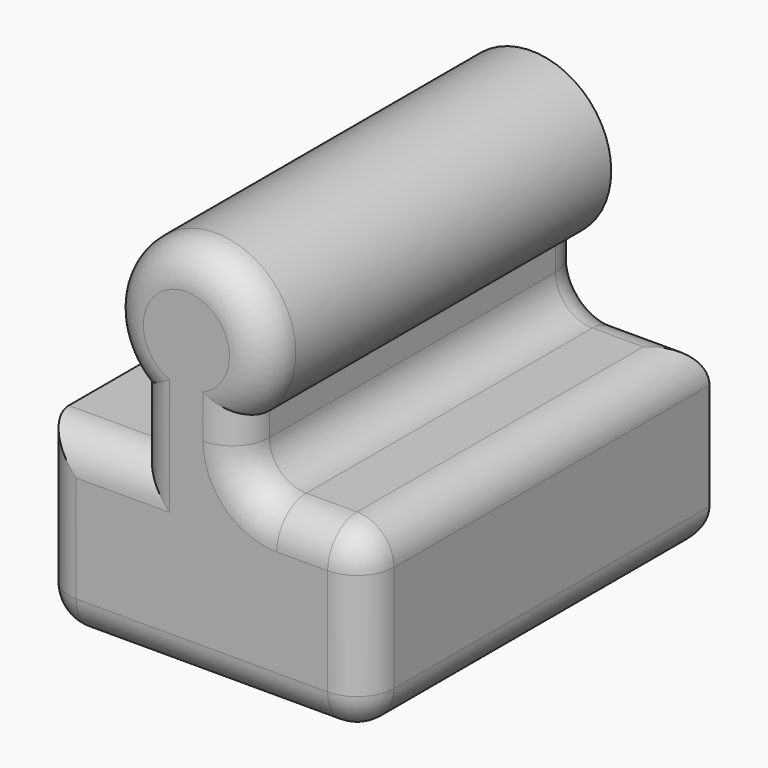
from build123d import *

# Parameters (mm, degrees)
F1_DEPTH = 179.578
F2_F1_R  = 15.3302561211
F2_F2_R  = 15.3302561211


with BuildPart() as f1:
    # F0 (on Front) → F1 (new body)
    with BuildSketch(Plane.XZ):
        with BuildLine():
            Line((-60.1250007749, 41.0845763981), (-99.0082323551, 41.0845763981))
            Line((-99.0082323551, 41.0845763981), (-99.0082323551, -33.9665971696))
            Line((-99.0082323551, -33.9665971696), (36.3630242646, -33.9665971696))
            Line((36.3630242646, -33.9665971696), (36.3630242646, 41.0845763981))
            Line((36.3630242646, 41.0845763981), (-15.4812876135, 41.0845763981))
            Line((-15.4812876135, 41.0845763981), (-15.4812876135, 66.3503706455))
            ThreePointArc((-15.4812876135, 66.3503706455), (-37.8031441942, 124.2664472866), (-60.1250007749, 66.3503706455))
            Line((-60.1250007749, 66.3503706455), (-60.1250007749, 41.0845763981))
        make_face()
    extrude(amount=F1_DEPTH)

    # F2: fillet of radius 15.3302561211 on 14 edges, made by hand

    # F2_f1
    f2_f1_edges = [f1.edges().sort_by_distance(p)[0] for p in [
        (-15.4812876135, -89.789, 41.0845763981),
    ]]
    fillet(f2_f1_edges, radius=F2_F1_R)

    # F2_f2
    f2_f2_edges = [f1.edges().sort_by_distance(p)[0] for p in [
        (36.3630242646, -89.789, 41.0845763981),
        (18.1059963861, 0, 41.0845763981),
        (18.1059963861, -179.578, 41.0845763981),
        (-99.0082323551, -89.789, -33.9665971696),
        (36.3630242646, -89.789, -33.9665971696),
        (-31.3226040453, 0, -33.9665971696),
        (-31.3226040453, -179.578, -33.9665971696),
        (-37.8031441942, -179.578, 124.2664472866),
        (-60.1250007749, -179.578, 53.7174735218),
        (-79.566616565, -179.578, 41.0845763981),
        (-99.0082323551, -179.578, 3.5589896142),
        (36.3630242646, -179.578, 3.5589896142),
        (-15.4812876135, -179.578, 61.3826015824),
        (-10.991159553, -179.578, 45.5747044587),
        (-10.991159553, 0, 45.5747044587),
    ]]
    fillet(f2_f2_edges, radius=F2_F2_R)


solid = f1.part
